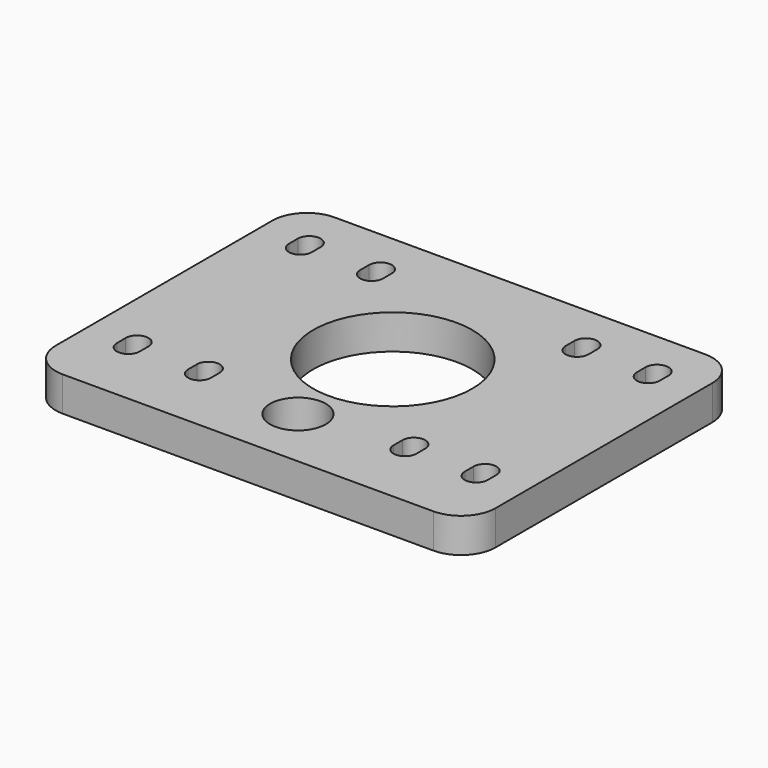
from build123d import *

# Parameters (mm, degrees)
F0_W     = 43
F0_H     = 46
F0_R     = 4.025
F0_R_2   = 11.5
F0_H_2   = 3.15
F1_DEPTH = 5
F2_R     = 5


# Not quite as in the source:
# - ends of sketch curves that miss each other by under 0.0002 mm in the source are joined


with BuildPart() as f1:
    # F0 (on Top) → F1 (new body)
    with BuildSketch(Plane.XY):
        Polygon((-21.5, -23), (-21.5, 23), (-31.8, 23), (-31.8, -26.15), (-21.5, -26.15), align=None)
        with BuildLine():
            ThreePointArc((-23.5, -16.35), (-25.15, -18), (-26.8, -16.35))
            Line((-26.8, -16.35), (-26.8, -14.75))
            ThreePointArc((-26.8, -14.75), (-25.15, -13.1), (-23.5, -14.75))
            Line((-23.5, -14.75), (-23.5, -16.35))
        make_face(mode=Mode.SUBTRACT)
        with BuildLine():
            ThreePointArc((-23.5, 14.75), (-25.15, 13.1), (-26.8, 14.75))
            Line((-26.8, 14.75), (-26.8, 16.35))
            ThreePointArc((-26.8, 16.35), (-25.15, 18), (-23.5, 16.35))
            Line((-23.5, 16.35), (-23.5, 14.75))
        make_face(mode=Mode.SUBTRACT)
        Rectangle(F0_W, F0_H)
        with BuildLine():
            ThreePointArc((-13.2000083949, -16.3447366346), (-13.2000020987, -16.3473683139), (-13.2, -16.35))
            ThreePointArc((-13.2, -16.35), (-14.85, -18), (-16.5, -16.35))
            Line((-16.5, -16.35), (-16.5, -14.75))
            ThreePointArc((-16.5, -14.75), (-14.8526316861, -13.1000020987), (-13.2000083949, -14.7447366346))
            ThreePointArc((-13.2000083949, -14.7447366346), (-13.2000020987, -14.7473683139), (-13.2, -14.75))
            Line((-13.2, -14.75), (-13.2000083949, -16.3447366346))
        make_face(mode=Mode.SUBTRACT)
        with Locations((0, -17.125)):
            Circle(F0_R, mode=Mode.SUBTRACT)
        with BuildLine():
            ThreePointArc((16.5, -16.35), (14.85, -18), (13.2, -16.35))
            Line((13.2, -16.35), (13.2, -14.75))
            ThreePointArc((13.2, -14.75), (14.85, -13.1), (16.5, -14.75))
            Line((16.5, -14.75), (16.5, -16.35))
        make_face(mode=Mode.SUBTRACT)
        with BuildLine():
            ThreePointArc((-16.5, 16.35), (-14.85, 18), (-13.2, 16.35))
            Line((-13.2, 16.35), (-13.2, 14.75))
            ThreePointArc((-13.2, 14.75), (-14.85, 13.1), (-16.5, 14.75))
            Line((-16.5, 14.75), (-16.5, 16.35))
        make_face(mode=Mode.SUBTRACT)
        Circle(F0_R_2, mode=Mode.SUBTRACT)
        with BuildLine():
            ThreePointArc((13.2, 16.35), (14.85, 18), (16.5, 16.35))
            ThreePointArc((16.5, 16.35), (16.4999973784, 16.347058674), (16.4999895135, 16.3441173573))
            Line((16.4999895135, 16.3441173573), (16.4999895135, 14.75))
            ThreePointArc((16.4999895135, 14.75), (14.85, 13.1), (13.2, 14.75))
            Line((13.2, 14.75), (13.2, 16.35))
        make_face(mode=Mode.SUBTRACT)
        with Locations((0, -24.575)):
            Rectangle(F0_W, F0_H_2)
        Polygon((31.7999895135, 23), (21.5, 23), (21.5, -23), (21.5, -26.15), (31.7999895135, -26.15), align=None)
        with BuildLine():
            ThreePointArc((26.8, -16.35), (25.15, -18), (23.5, -16.35))
            Line((23.5, -16.35), (23.5, -14.75))
            ThreePointArc((23.5, -14.75), (25.15, -13.1), (26.8, -14.75))
            Line((26.8, -14.75), (26.8, -16.35))
        make_face(mode=Mode.SUBTRACT)
        with BuildLine():
            ThreePointArc((26.7999895135, 14.75), (25.1499895135, 13.1), (23.4999895135, 14.75))
            Line((23.4999895135, 14.75), (23.4999895135, 16.3441173573))
            ThreePointArc((23.4999895135, 16.3441173573), (25.1499895135, 17.9941173573), (26.7999895135, 16.3441173573))
            Line((26.7999895135, 16.3441173573), (26.7999895135, 14.75))
        make_face(mode=Mode.SUBTRACT)
    extrude(amount=F1_DEPTH)

    # F2
    f2_edges = [f1.edges().sort_by_distance(p)[0] for p in [
        (-31.8, 23, 2.5),
        (-31.8, -26.15, 2.5),
        (31.79999, -26.15, 2.5),
        (31.79999, 23, 2.5),
    ]]
    fillet(f2_edges, radius=F2_R)


solid = f1.part
